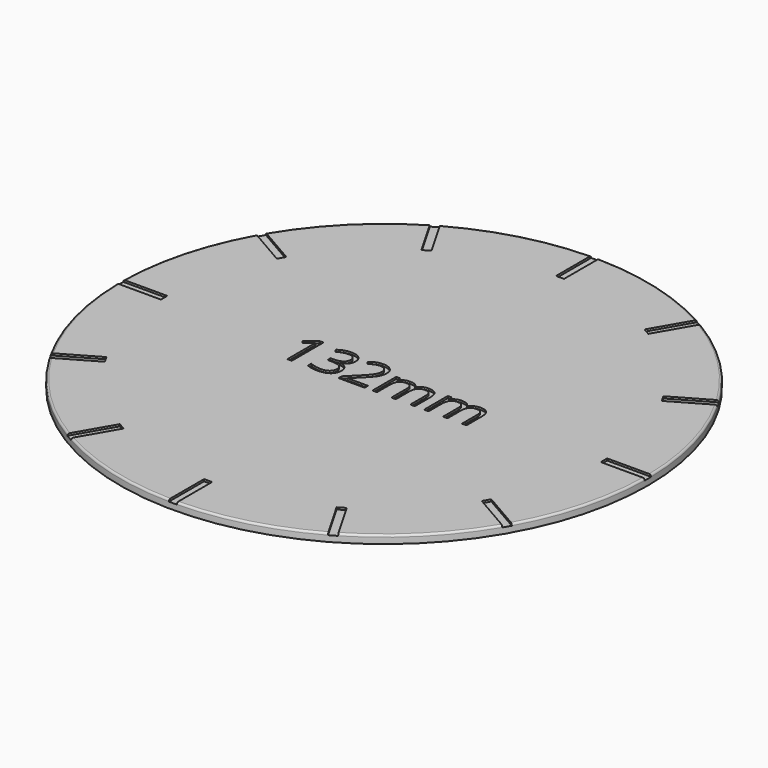
from build123d import *

# Parameters (mm, degrees)
F0_R         = 66
F1_DEPTH     = 2
F2_W         = 2
F2_H         = 15
F2_W_2       = 15
F2_H_2       = 2
F3_DEPTH     = 0.5
F4_TEXT_SIZE = 13.888889872
F5_DEPTH     = 0.5
F6_R         = 0.5


# Not quite as in the source:
# - Text() gives the source's letters only with a copy of the font that has no kerning and outlines rounded to 1/6400 em; it was checked with that copy


with BuildPart() as f1:
    # F0 (on Top) → F1 (new body)
    with BuildSketch(Plane.XY):
        Circle(F0_R)
    extrude(amount=F1_DEPTH)

    # F2 (on face) → F3 (cut)
    with BuildSketch(Plane.XY.offset(2)):
        with Locations((0, 62.5)):
            Rectangle(F2_W, F2_H)
        Polygon((-34.1339745962, 61.1217782649), (-35.8660254038, 60.1217782649), (-28.3660254038, 47.1313972081), (-26.6339745962, 48.1313972081), align=None)
        Polygon((-60.1217782649, 35.8660254038), (-61.1217782649, 34.1339745962), (-48.1313972081, 26.6339745962), (-47.1313972081, 28.3660254038), align=None)
        with Locations((-62.5, 0)):
            Rectangle(F2_W_2, F2_H_2)
        Polygon((-61.1217782649, -34.1339745962), (-60.1217782649, -35.8660254038), (-47.1313972081, -28.3660254038), (-48.1313972081, -26.6339745962), align=None)
        Polygon((-35.8660254038, -60.1217782649), (-34.1339745962, -61.1217782649), (-26.6339745962, -48.1313972081), (-28.3660254038, -47.1313972081), align=None)
        with Locations((0, -62.5)):
            Rectangle(F2_W, F2_H)
        Polygon((34.1339745962, -61.1217782649), (35.8660254038, -60.1217782649), (28.3660254038, -47.1313972081), (26.6339745962, -48.1313972081), align=None)
        Polygon((60.1217782649, -35.8660254038), (61.1217782649, -34.1339745962), (48.1313972081, -26.6339745962), (47.1313972081, -28.3660254038), align=None)
        with Locations((62.5, 0)):
            Rectangle(F2_W_2, F2_H_2)
        Polygon((61.1217782649, 34.1339745962), (60.1217782649, 35.8660254038), (47.1313972081, 28.3660254038), (48.1313972081, 26.6339745962), align=None)
        Polygon((35.8660254038, 60.1217782649), (34.1339745962, 61.1217782649), (26.6339745962, 48.1313972081), (28.3660254038, 47.1313972081), align=None)
    extrude(amount=-F3_DEPTH, mode=Mode.SUBTRACT)

    # F4 (on face) → F5 (cut)
    with BuildSketch(Plane.XY.offset(2)):
        with Locations((-23.7285758194, -5.2462602034)):
            Text('132mm', F4_TEXT_SIZE, font='Open Sans', text_align=(TextAlign.LEFT, TextAlign.BOTTOM))
    extrude(amount=-F5_DEPTH, mode=Mode.SUBTRACT)

    # F6
    f6_edges = [f1.edges().sort_by_distance(p)[0] for p in [
        (46.669048, 46.669048, 2),
        (63.751105, 17.082057, 2),
        (63.751105, -17.082057, 2),
        (46.669048, -46.669048, 2),
        (17.082057, -63.751105, 2),
        (-17.082057, -63.751105, 2),
        (-46.669048, -46.669048, 2),
        (-63.751105, -17.082057, 2),
        (-63.751105, 17.082057, 2),
        (-46.669048, 46.669048, 2),
        (-17.082057, 63.751105, 2),
        (17.082057, 63.751105, 2),
    ]]
    fillet(f6_edges, radius=F6_R)


solid = f1.part
